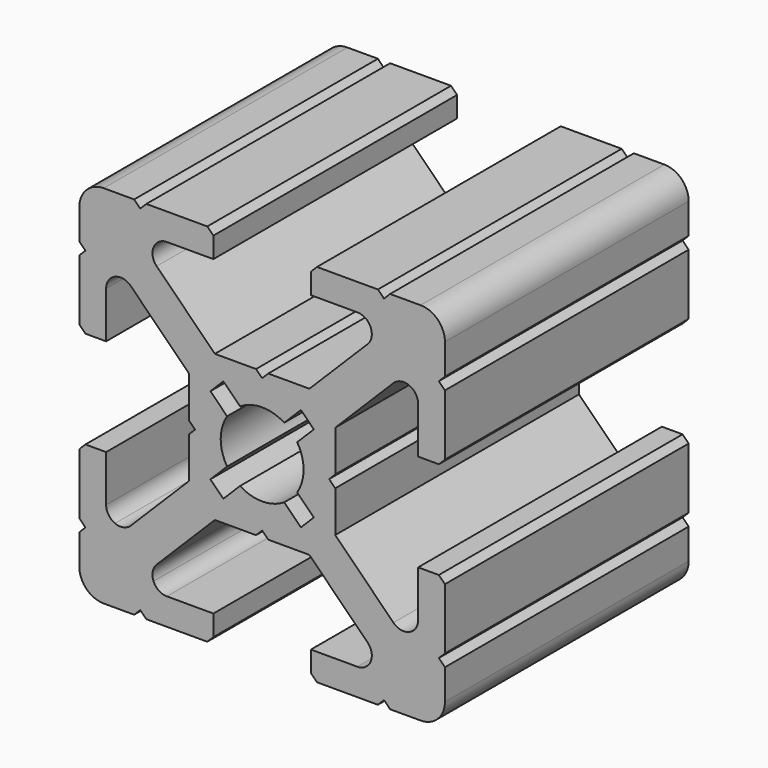
from build123d import *

# Parameters (mm, degrees)
F1_DEPTH = 25


# Not quite as in the source:
# - ends of sketch curves that miss each other by under 0.0002 mm in the source are joined


with BuildPart() as f1:
    # F0 (on Front) → F1 (new body)
    with BuildSketch(Plane.XZ):
        with BuildLine():
            ThreePointArc((-12.0672760652, 8.9096491574), (-11.3814883912, 8.9771930389), (-10.7737513132, 8.6523506868))
            Line((-10.7737513132, 8.6523506868), (-6, 3.8786))
            Line((-6, 3.8786), (-6, 0.5))
            Line((-6, 0.5), (-5.5, 0))
            Line((-5.5, 0), (-6, -0.5))
            Line((-6, -0.5), (-6, -3.8786))
            Line((-6, -3.8786), (-10.7738, -8.6524))
            ThreePointArc((-10.7738, -8.6524), (-11.3814883912, -8.9771930389), (-12.0672760652, -8.9096491574))
            ThreePointArc((-12.0672760652, -8.9096491574), (-12.5999492171, -8.4725051968), (-12.799999999, -7.8131))
            Line((-12.799999999, -7.8131), (-12.8, -4))
            Line((-12.8, -4), (-14.5, -4))
            Line((-14.5, -4), (-15, -4.5))
            Line((-15, -4.5), (-15, -9.5))
            Line((-15, -9.5), (-14.5, -10))
            Line((-14.5, -10), (-15, -10.5))
            Line((-15, -10.5), (-15, -13))
            ThreePointArc((-15, -13), (-14.4141844722, -14.4142216524), (-13, -15.0000239995))
            Line((-13, -15.0000239995), (-10.5, -15))
            Line((-10.5, -15), (-10, -14.5))
            Line((-10, -14.5), (-9.5, -15))
            Line((-9.5, -15), (-4.5, -15))
            Line((-4.5, -15), (-4, -14.5))
            Line((-4, -14.5), (-4, -12.8))
            Line((-4, -12.8), (-7.8131, -12.8))
            ThreePointArc((-7.8131, -12.8), (-8.4725048128, -12.5999494737), (-8.9096488038, -12.0672769187))
            ThreePointArc((-8.9096488038, -12.0672769187), (-8.977199798, -11.3815223738), (-8.6523996854, -10.7738003146))
            Line((-8.6523996854, -10.7738003146), (-3.8786, -6))
            Line((-3.8786, -6), (-0.5, -6))
            Line((-0.5, -6), (0, -5.5))
            Line((0, -5.5), (0.5, -6))
            Line((0.5, -6), (3.8786, -6))
            Line((3.8786, -6), (8.6524, -10.7738))
            ThreePointArc((8.6524, -10.7738), (8.977199798, -11.3815223738), (8.9096491574, -12.0672760652))
            ThreePointArc((8.9096491574, -12.0672760652), (8.4725048128, -12.5999494737), (7.8131, -12.799999999))
            Line((7.8131, -12.799999999), (4, -12.8))
            Line((4, -12.8), (4, -14.5))
            Line((4, -14.5), (4.5, -15))
            Line((4.5, -15), (9.5, -15))
            Line((9.5, -15), (10, -14.5))
            Line((10, -14.5), (10.5, -15))
            Line((10.5, -15), (13, -15))
            ThreePointArc((13, -15), (14.4141844722, -14.4142216524), (14.999955, -13.000024))
            Line((14.999955, -13.000024), (15, -10.5))
            Line((15, -10.5), (14.5, -10))
            Line((14.5, -10), (15, -9.5))
            Line((15, -9.5), (15, -4.5))
            Line((15, -4.5), (14.5, -4))
            Line((14.5, -4), (12.8, -4))
            Line((12.8, -4), (12.8, -7.8131))
            ThreePointArc((12.8, -7.8131), (12.5999492171, -8.4725051968), (12.0672760652, -8.9096491574))
            ThreePointArc((12.0672760652, -8.9096491574), (11.3814883912, -8.9771930389), (10.7737513132, -8.6523506868))
            Line((10.7737513132, -8.6523506868), (6, -3.8786))
            Line((6, -3.8786), (6, -0.5))
            Line((6, -0.5), (5.5, 0))
            Line((5.5, 0), (6, 0.5))
            Line((6, 0.5), (6, 3.8786))
            Line((6, 3.8786), (10.7738, 8.6524))
            ThreePointArc((10.7738, 8.6524), (11.3814883912, 8.9771930389), (12.0672760652, 8.9096491574))
            ThreePointArc((12.0672760652, 8.9096491574), (12.5999492171, 8.4725051968), (12.799999999, 7.8131))
            Line((12.799999999, 7.8131), (12.8, 4))
            Line((12.8, 4), (14.5, 4))
            Line((14.5, 4), (15, 4.5))
            Line((15, 4.5), (15, 9.5))
            Line((15, 9.5), (14.5, 10))
            Line((14.5, 10), (15, 10.5))
            Line((15, 10.5), (15, 13))
            ThreePointArc((15, 13), (14.4141844722, 14.4142216524), (13, 15.0000239995))
            Line((13, 15.0000239995), (10.5, 15))
            Line((10.5, 15), (10, 14.5))
            Line((10, 14.5), (9.5, 15))
            Line((9.5, 15), (4.5, 15))
            Line((4.5, 15), (4, 14.5))
            Line((4, 14.5), (4, 12.8))
            Line((4, 12.8), (7.8131, 12.8))
            ThreePointArc((7.8131, 12.8), (8.4725048128, 12.5999494737), (8.9096488038, 12.0672769187))
            ThreePointArc((8.9096488038, 12.0672769187), (8.977199798, 11.3815223738), (8.6523996854, 10.7738003146))
            Line((8.6523996854, 10.7738003146), (3.8786, 6))
            Line((3.8786, 6), (0.5, 6))
            Line((0.5, 6), (0, 5.5))
            Line((0, 5.5), (-0.5, 6))
            Line((-0.5, 6), (-3.8786, 6))
            Line((-3.8786, 6), (-8.6524, 10.7738))
            ThreePointArc((-8.6524, 10.7738), (-8.977199798, 11.3815223738), (-8.9096491574, 12.0672760652))
            ThreePointArc((-8.9096491574, 12.0672760652), (-8.4725048128, 12.5999494737), (-7.8131, 12.799999999))
            Line((-7.8131, 12.799999999), (-4, 12.8))
            Line((-4, 12.8), (-4, 14.5))
            Line((-4, 14.5), (-4.5, 15))
            Line((-4.5, 15), (-9.5, 15))
            Line((-9.5, 15), (-10, 14.5))
            Line((-10, 14.5), (-10.5, 15))
            Line((-10.5, 15), (-13, 15))
            ThreePointArc((-13, 15), (-14.4141844722, 14.4142216524), (-14.999955, 13.000024))
            Line((-14.999955, 13.000024), (-15, 10.5))
            Line((-15, 10.5), (-14.5, 10))
            Line((-14.5, 10), (-15, 9.5))
            Line((-15, 9.5), (-15, 4.5))
            Line((-15, 4.5), (-14.5, 4))
            Line((-14.5, 4), (-12.8, 4))
            Line((-12.8, 4), (-12.8, 7.8131))
            ThreePointArc((-12.8, 7.8131), (-12.5999492171, 8.4725051968), (-12.0672760652, 8.9096491574))
        make_face()
        with BuildLine():
            Line((-4.2426, -3.182), (-2.8752, -1.8146))
            ThreePointArc((-2.8752, -1.8146), (-3.4, 0), (-2.8752481958, 1.8146481236))
            Line((-2.8752481958, 1.8146481236), (-4.2426, 3.182))
            Line((-4.2426, 3.182), (-3.182, 4.2426))
            Line((-3.182, 4.2426), (-1.8146, 2.8752))
            ThreePointArc((-1.8146, 2.8752), (0, 3.4), (1.8146481236, 2.8752481958))
            Line((1.8146481236, 2.8752481958), (3.182, 4.2426))
            Line((3.182, 4.2426), (4.2426, 3.182))
            Line((4.2426, 3.182), (2.8752, 1.8146))
            ThreePointArc((2.8752, 1.8146), (3.4, 0), (2.8752481958, -1.8146481236))
            Line((2.8752481958, -1.8146481236), (4.2426, -3.182))
            Line((4.2426, -3.182), (3.182, -4.2426))
            Line((3.182, -4.2426), (1.8146, -2.8752))
            ThreePointArc((1.8146, -2.8752), (0, -3.4), (-1.8146481236, -2.8752481958))
            Line((-1.8146481236, -2.8752481958), (-3.182, -4.2426))
            Line((-3.182, -4.2426), (-4.2426, -3.182))
        make_face(mode=Mode.SUBTRACT)
    extrude(amount=F1_DEPTH)


solid = f1.part
